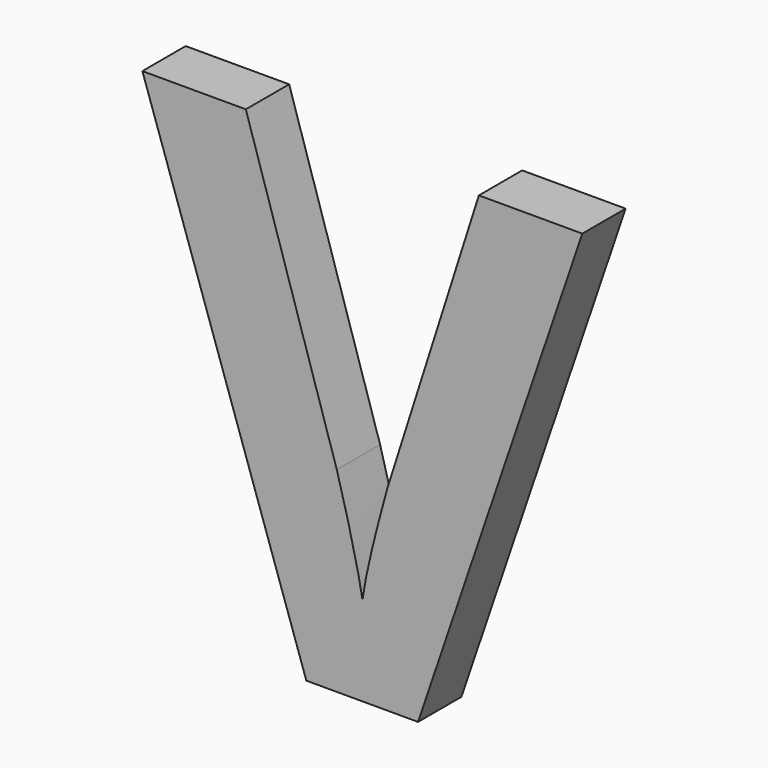
from build123d import *

# Parameters (mm, degrees)
F0_TEXT_SIZE = 62.5
F1_DEPTH     = 5


# Not quite as in the source:
# - Text() gives the source's letters only with a copy of the font that has no kerning and outlines rounded to 1/6400 em; it was checked with that copy


with BuildPart() as f1:
    # F0 (on Front) → F1 (new body)
    with BuildSketch(Plane.XZ):
        with Locations((-57.7016074898, 15.7258056963)):
            Text('V', F0_TEXT_SIZE, font='Open Sans', font_style=FontStyle.BOLD, text_align=(TextAlign.LEFT, TextAlign.BOTTOM))
    extrude(amount=F1_DEPTH)


solid = f1.part
